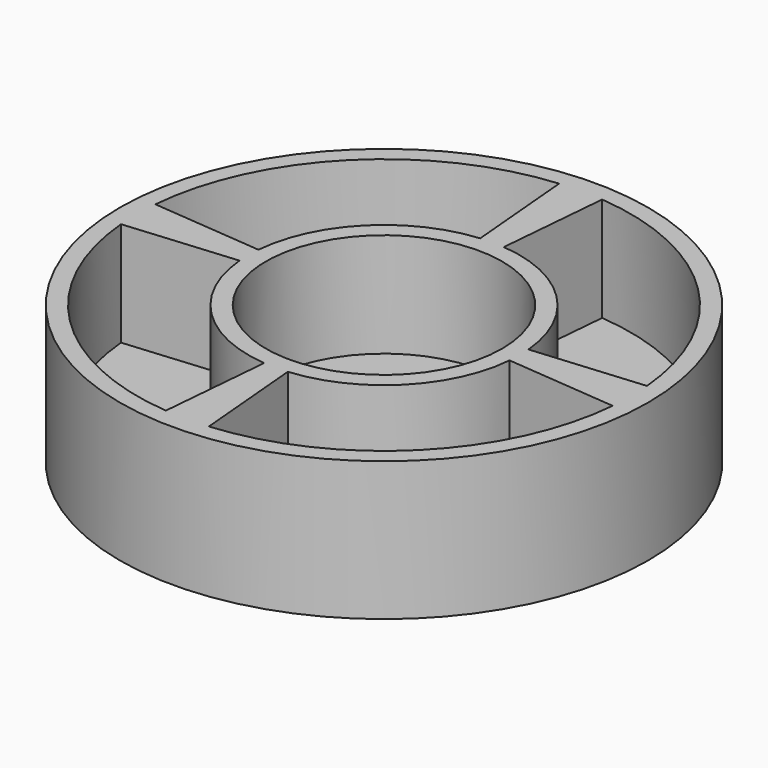
from build123d import *

# Parameters (mm, degrees)
F0_R         = 38
F1_DEPTH     = 20
F2_R         = 17
F3_DEPTH     = 15
F4_TEXT_SIZE = 15.0948482092
F5_DEPTH     = 2


# Not quite as in the source:
# - Text() gives the source's letters only with a copy of the font that has no kerning and outlines rounded to 1/6400 em; it was checked with that copy


with BuildPart() as f1:
    # F0 (on Top) → F1 (new body)
    with BuildSketch(Plane.XY):
        Circle(F0_R)
    extrude(amount=F1_DEPTH)

    # F2 (on face) → F3 (cut)
    with BuildSketch(Plane.XY.offset(20)):
        with BuildLine():
            Line((-1.6995369836, 19.4257966128), (-3.0940288675, 35.3649117823))
            ThreePointArc((-3.0940288675, 35.3649117823), (-25.1022907321, 25.1022907321), (-35.3649117823, 3.0940288675))
            Line((-35.3649117823, 3.0940288675), (-19.4257966128, 1.6995369836))
            ThreePointArc((-19.4257966128, 1.6995369836), (-13.7885822331, 13.7885822331), (-1.6995369836, 19.4257966128))
        make_face()
        with BuildLine():
            Line((3.0940288675, 35.3649117823), (1.6995369836, 19.4257966128))
            ThreePointArc((1.6995369836, 19.4257966128), (13.7885822331, 13.7885822331), (19.4257966128, 1.6995369836))
            Line((19.4257966128, 1.6995369836), (35.3649117823, 3.0940288675))
            ThreePointArc((35.3649117823, 3.0940288675), (25.1022907321, 25.1022907321), (3.0940288675, 35.3649117823))
        make_face()
        with BuildLine():
            ThreePointArc((-1.6995369836, -19.4257966128), (-13.7885822331, -13.7885822331), (-19.4257966128, -1.6995369836))
            Line((-19.4257966128, -1.6995369836), (-35.3649117823, -3.0940288675))
            ThreePointArc((-35.3649117823, -3.0940288675), (-25.1022907321, -25.1022907321), (-3.0940288675, -35.3649117823))
            Line((-3.0940288675, -35.3649117823), (-1.6995369836, -19.4257966128))
        make_face()
        with BuildLine():
            Line((1.6995369836, -19.4257966128), (3.0940288675, -35.3649117823))
            ThreePointArc((3.0940288675, -35.3649117823), (25.1022907321, -25.1022907321), (35.3649117823, -3.0940288675))
            Line((35.3649117823, -3.0940288675), (19.4257966128, -1.6995369836))
            ThreePointArc((19.4257966128, -1.6995369836), (13.7885822331, -13.7885822331), (1.6995369836, -19.4257966128))
        make_face()
        Circle(F2_R)
    extrude(amount=-F3_DEPTH, mode=Mode.SUBTRACT)

    # F4 (on face) → F5 (cut)
    with BuildSketch(Plane(origin=(0, 0, 0), x_dir=(1, 0, 0), z_dir=(0, 0, -1))):
        with Locations((-34.8796120487, -5.2811949803)):
            Text('Footbutts', F4_TEXT_SIZE, font='Arimo', font_style=FontStyle.BOLD, text_align=(TextAlign.LEFT, TextAlign.BOTTOM))
    extrude(amount=-F5_DEPTH, mode=Mode.SUBTRACT)


solid = f1.part
